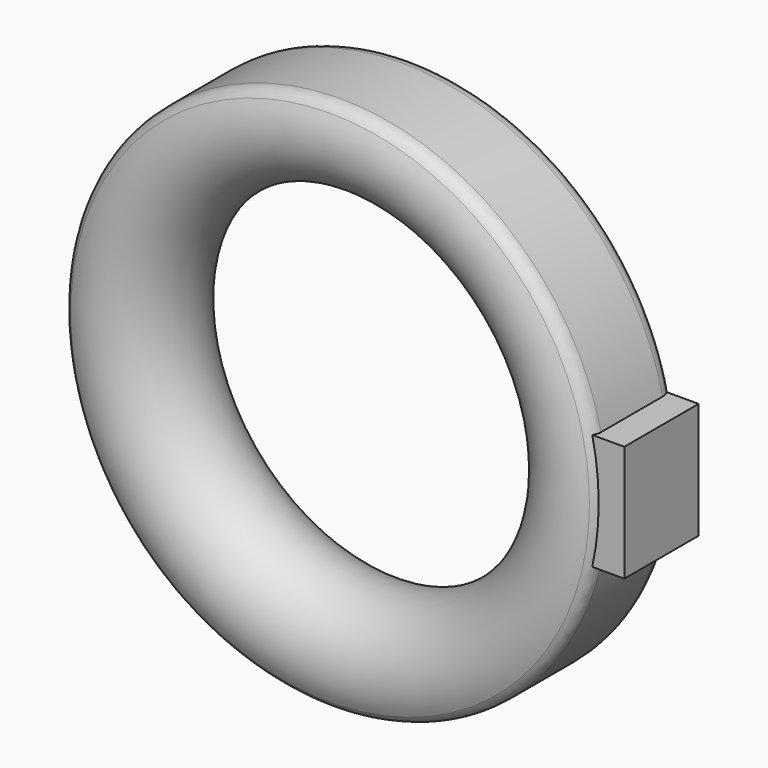
from build123d import *

# Parameters (mm, degrees)
F2_R     = 0.79375
F3_W     = 1.905
F3_H     = 5.08
F4_DEPTH = 3.175


with BuildPart() as f1:
    # F0 (on Top) → F1 (revolve)
    with BuildSketch(Plane.XY):
        with BuildLine():
            Line((14.605, -2.54), (14.605, 2.54))
            ThreePointArc((14.605, 2.54), (9.525, 0), (14.605, -2.54))
        make_face()
    revolve(axis=Axis((0, 7.2536539203, 0), (0, 1, 0)))

    # F2
    f2_edges = [f1.edges().sort_by_distance(p)[0] for p in [
        (-14.605, 2.54, 0),
        (-14.605, -2.54, 0),
    ]]
    fillet(f2_edges, radius=F2_R)

    # F3 (on Top) → F4 (join, symmetric)
    with BuildSketch(Plane.XY):
        with Locations((14.9225, 0)):
            Rectangle(F3_W, F3_H)
    extrude(amount=F4_DEPTH, both=True)


solid = f1.part
